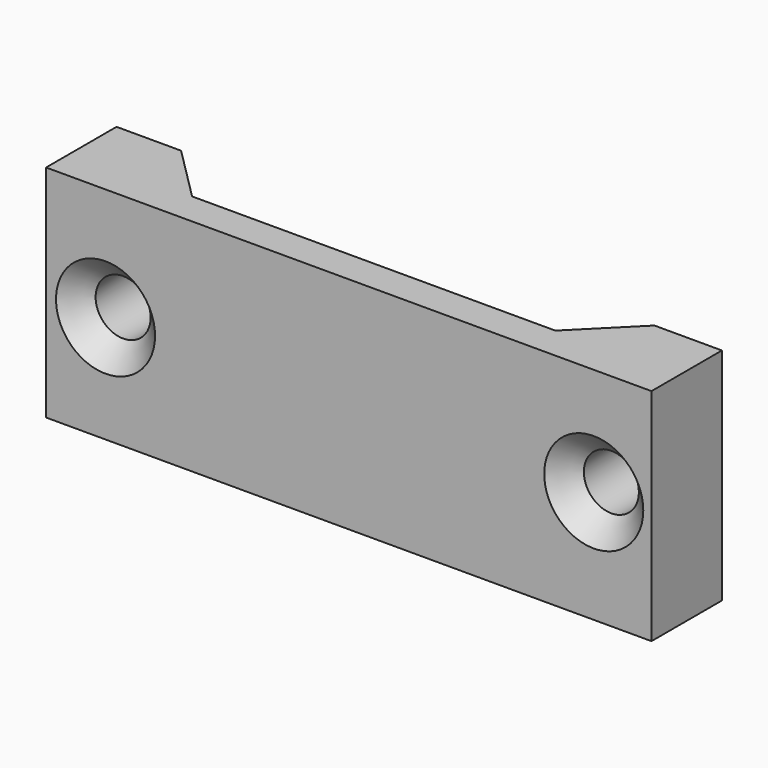
from build123d import *

# Parameters (mm, degrees)
F0_W        = 55
F0_H        = 8
F1_DEPTH    = 20
F2_R        = 2.5
F3_DEPTH    = 35.3
F4_W        = 33
F4_H        = 86
F5_DEPTH    = 5
F6_SIZE     = 2
F7_SIZE     = 2
F8_T4_DEPTH = 45.7168298797
F8_T9_DEPTH = 45.7168298797


# Not quite as in the source:
# - a fillet or chamfer that OpenCascade refuses, or shapes differently, is made with other operations: its cross-section is extruded or revolved along the edge and cut away or added


with BuildPart() as f1:
    # F0 (on Top) → F1 (new body)
    with BuildSketch(Plane.XY):
        with Locations((-34.4500018656, -4)):
            Rectangle(F0_W, F0_H)
    extrude(amount=F1_DEPTH)

    # F2 (on Front) → F3 (cut)
    with BuildSketch(Plane.XZ):
        with Locations((-56.5492250025, 9.7595239058)):
            Circle(F2_R)
        with Locations((-12.1940001845, 10.2066537365)):
            Circle(F2_R)
    extrude(amount=F3_DEPTH, mode=Mode.SUBTRACT)

    # F4 (on Front) → F5 (cut)
    with BuildSketch(Plane.XZ):
        with Locations((-34.5833339691, 26.0833319575)):
            Rectangle(F4_W, F4_H)
    extrude(amount=F5_DEPTH, mode=Mode.SUBTRACT)

    # F6
    f6_edges = [f1.edges().sort_by_distance(p)[0] for p in [
        (-14.694, -8, 10.206654),
    ]]
    chamfer(f6_edges, length=F6_SIZE)

    # F7
    f7_edges = [f1.edges().sort_by_distance(p)[0] for p in [
        (-59.049225, -8, 9.759524),
    ]]
    chamfer(f7_edges, length=F7_SIZE)

    # F8: chamfer of 5 on 2 edges, made by hand


with BuildPart() as f8_tool2:
    # F8_s3 → F8_t4 (new body)
    with BuildSketch(Plane.XY.offset(32.8584149398)):
        Polygon((-56.0833339691, 0), (-51.0833339691, -5), (-51.0833339691, 0), align=None)
    extrude(amount=-F8_T4_DEPTH)

    split(bisect_by=Plane.XZ.offset(5), keep=Keep.BOTTOM)


with BuildPart() as f1_1:
    add(f1.part)

    # F8_t1: cut F8_tool2
    add(f8_tool2.part, mode=Mode.SUBTRACT)


with BuildPart() as f8_tool7:
    # F8_s8 → F8_t9 (new body)
    with BuildSketch(Plane.XY.offset(-12.8584149398)):
        Polygon((-18.0833339691, -5), (-13.0833339691, 0), (-18.0833339691, 0), align=None)
    extrude(amount=F8_T9_DEPTH)

    split(bisect_by=Plane.XZ.offset(5), keep=Keep.BOTTOM)


with BuildPart() as f1_2:
    add(f1_1.part)

    # F8_t6: cut F8_tool7
    add(f8_tool7.part, mode=Mode.SUBTRACT)


solid = f1_2.part
